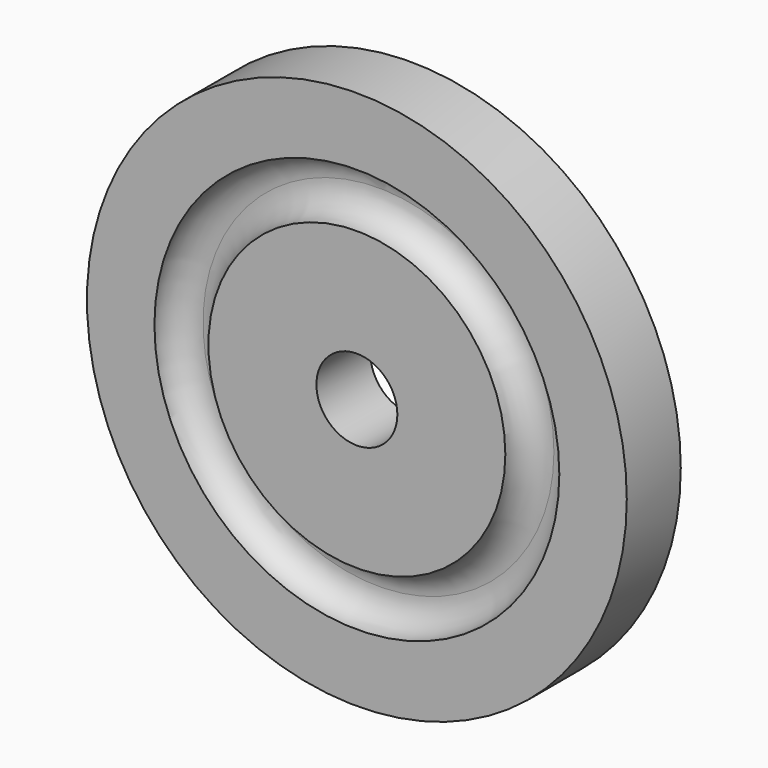
from build123d import *

# Parameters (mm, degrees)
F0_R     = 25.4
F0_R_2   = 3.81
F1_DEPTH = 6.35
F2_R     = 19.05
F2_R_2   = 13.97
F3_DEPTH = 2.54
F4_R     = 2.53999


# Not quite as in the source:
# - a fillet or chamfer is up to 0.001 mm smaller than in the source, because OpenCascade refuses the exact size


with BuildPart() as f1:
    # F0 (on Front) → F1 (new body)
    with BuildSketch(Plane.XZ):
        Circle(F0_R)
        Circle(F0_R_2, mode=Mode.SUBTRACT)
    extrude(amount=F1_DEPTH)

    # F2 (on face) → F3 (cut)
    with BuildSketch(Plane.XZ.offset(6.35)):
        Circle(F2_R)
        Circle(F2_R_2, mode=Mode.SUBTRACT)
    extrude(amount=-F3_DEPTH, mode=Mode.SUBTRACT)

    # F4 (radius 2.54 in the source; OpenCascade refuses exactly that, so slightly less here)
    f4_edges = [f1.edges().sort_by_distance(p)[0] for p in [
        (-19.05, -3.81, 0),
        (-13.97, -3.81, 0),
    ]]
    fillet(f4_edges, radius=F4_R)


solid = f1.part
